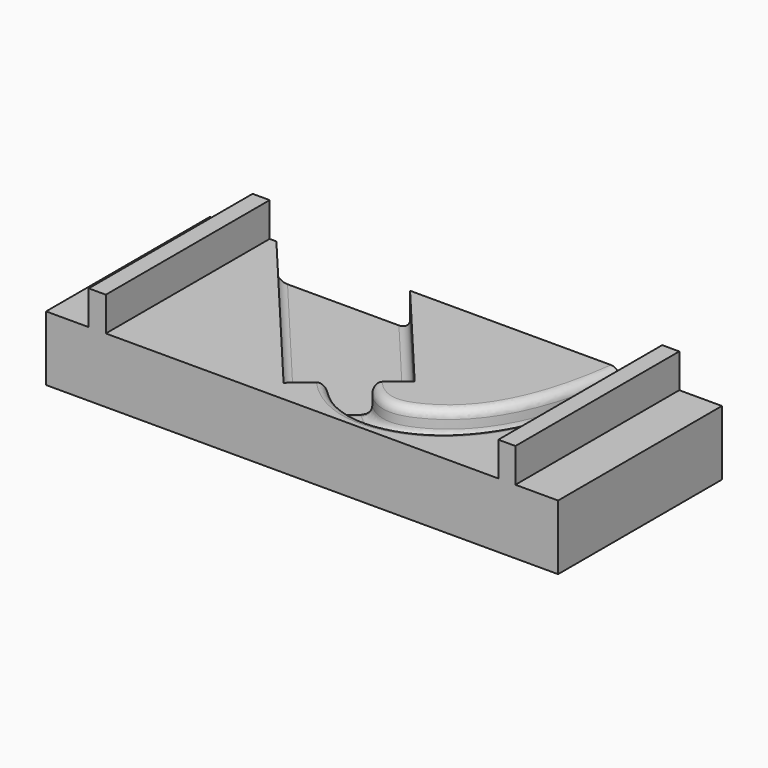
from build123d import *

# Parameters (mm, degrees)
F0_W     = 30
F0_H     = 12
F1_DEPTH = 3.8
F2_W     = 1
F2_H     = 12
F3_DEPTH = 2
F4_DEPTH = 2
F5_DEPTH = 1.5
F6_F1_R  = 0.5
F6_F2_R  = 0.4999


# Not quite as in the source:
# - a fillet or chamfer is up to 0.001 mm smaller than in the source, because OpenCascade refuses the exact size


with BuildPart() as f1:
    # F0 (on Top) → F1 (new body)
    with BuildSketch(Plane.XY):
        with Locations((15, -6)):
            Rectangle(F0_W, F0_H)
    extrude(amount=F1_DEPTH)

    # F2 (on face) → F3 (join)
    with BuildSketch(Plane.XY.offset(3.8)):
        with Locations((3, -6)):
            Rectangle(F2_W, F2_H)
        with Locations((27, -6)):
            Rectangle(F2_W, F2_H)
    extrude(amount=F3_DEPTH)

    # F2 (on face) → F4 (cut)
    with BuildSketch(Plane.XY.offset(3.8)):
        Polygon((11.7273407389, 0), (3.8948970029, 0), (12.9037333413, -10.7363130714), (14.4358222275, -9.450737852), (15.9679111138, -8.1651626326), (17.5, -6.8795874133), align=None)
    extrude(amount=-F4_DEPTH, mode=Mode.SUBTRACT)

    # F2 (on face) → F5 (cut)
    with BuildSketch(Plane.XY.offset(3.8)):
        with BuildLine():
            Line((15.9679111138, -8.1651626326), (14.4358222275, -9.450737852))
            add(Edge.make_bspline(
                [(14.4358222275, -9.450737852), (15.863483823, -11.0007241913), (20.1732023491, -12.1940239487), (24.8259473592, -7.8065069392), (25.5, 0)],
                knots=[0, 0, 0, 0, 0.3873861913, 1, 1, 1, 1], degree=3))
            Line((25.5, 0), (24, 0))
            add(Edge.make_bspline(
                [(15.9679111138, -8.1651626326), (17.165783315, -9.5028725168), (20.0701277214, -9.1607729948), (23.2835721894, -5.7138572024), (24, 0)],
                knots=[0, 0, 0, 0, 0.3706088241, 1, 1, 1, 1], degree=3))
        make_face()
    extrude(amount=-F5_DEPTH, mode=Mode.SUBTRACT)

    # F6: fillet of radius 0.5 on 7 edges, made by hand

    # F6_f1
    f6_f1_edges = [f1.edges().sort_by_distance(p)[0] for p in [
        (20.5359596674, -8.067345607, 2.3),
        (20.7536395384, -10.5294024966, 2.3),
        (14.6136703694, -3.4397937066, 1.8),
        (8.3993151721, -5.3681565357, 1.8),
    ]]
    fillet(f6_f1_edges, radius=F6_F1_R)

    # F6_f2 (radius 0.5 in the source; OpenCascade refuses exactly that, so slightly less here)
    f6_f2_edges = [f1.edges().sort_by_distance(p)[0] for p in [
        (20.5359596674, -8.067345607, 3.8),
        (20.7536395384, -10.5294024966, 3.8),
        (15.9679111138, -8.1651626326, 3.3),
        (15.8556697669, -8.2593443054, 2.446446382),
    ]]
    fillet(f6_f2_edges, radius=F6_F2_R)


solid = f1.part
